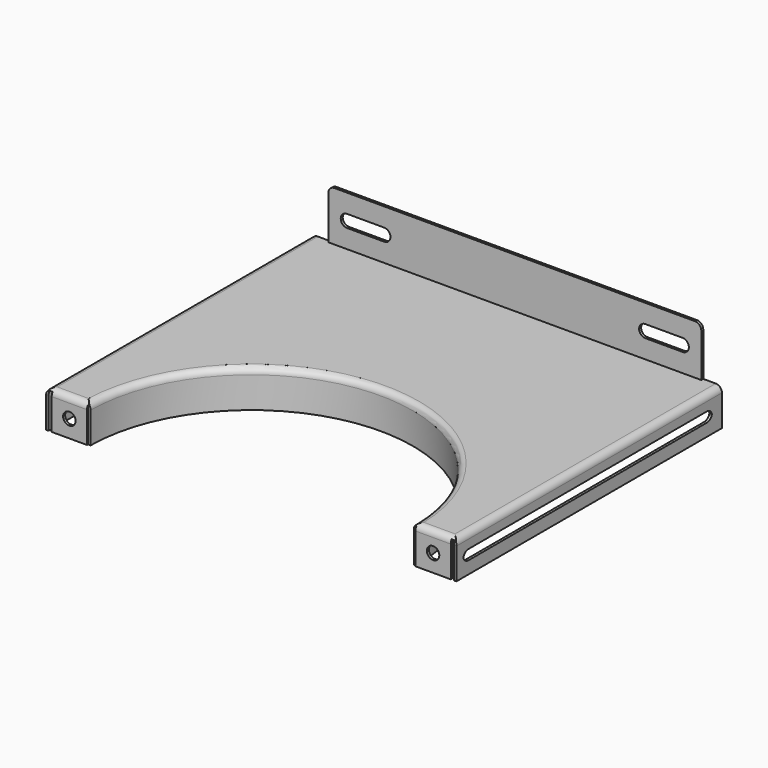
from build123d import *

# Parameters (mm, degrees)
F1_DEPTH       = 267
F2_W           = 250
F2_H           = 8
F3_DEPTH       = 5
F4_R           = 130
F5_DEPTH       = 12.5
F6_W           = 150
F6_H           = 40
F7_DEPTH       = 2
F8_W           = 40
F8_H           = 10
F9_DEPTH       = 12.5
F10_F1_R       = 5
F10_F2_R       = 5
F10_F3_R       = 4.9999
F10_F4_R       = 4.9999
F10_2_T1_DEPTH = 35
F11_W          = 28.4319519997
F11_H          = 28
F12_DEPTH      = 2
F13_R          = 5
F14_DEPTH      = 5
F17_T1_DEPTH   = 27
F17_T3_DEPTH   = 292
F17_T5_DEPTH   = 60
F20_DEPTH      = 28
F21_T2_ANGLE   = 186.62682558


# Not quite as in the source:
# - a fillet or chamfer that OpenCascade refuses, or shapes differently, is made with other operations: its cross-section is extruded or revolved along the edge and cut away or added
# - a fillet or chamfer is up to 0.001 mm smaller than in the source, because OpenCascade refuses the exact size


with BuildPart() as f1:
    # F0 (on Front) → F1 (new body)
    with BuildSketch(Plane.XZ):
        Polygon((-165, -30), (-163, -30), (-163, -2), (0, -2), (0, 0), (-165, 0), align=None)
    extrude(amount=F1_DEPTH)


with BuildPart() as f3:
    # F2 (on face) → F3 (new body, symmetric)
    with BuildSketch(Plane(origin=(-165, 0, 0), x_dir=(0, -1, 0), z_dir=(-1, 0, 0))):
        with Locations((135, -16)):
            Rectangle(F2_W, F2_H)
    extrude(amount=F3_DEPTH, both=True)

    # F10#2: fillet of radius 5 on 4 edges, made by hand

    # F10_2_s2 → F10_2_t1 (cut)
    with BuildSketch(Plane.YZ.offset(-182.5)):
        with BuildLine():
            ThreePointArc((-15, -12), (-11.4644660941, -13.4644660941), (-10, -17))
            Line((-10, -17), (-10, -12))
            Line((-10, -12), (-15, -12))
        make_face()
        with BuildLine():
            ThreePointArc((-15, -20), (-11.4644660941, -18.5355339059), (-10, -15))
            Line((-10, -15), (-10, -20))
            Line((-10, -20), (-15, -20))
        make_face()
        with BuildLine():
            ThreePointArc((-260, -15), (-258.5355339059, -18.5355339059), (-255, -20))
            Line((-255, -20), (-260, -20))
            Line((-260, -20), (-260, -15))
        make_face()
        with BuildLine():
            ThreePointArc((-255, -12), (-258.5355339059, -13.4644660941), (-260, -17))
            Line((-260, -17), (-260, -12))
            Line((-260, -12), (-255, -12))
        make_face()
    extrude(amount=F10_2_T1_DEPTH, mode=Mode.SUBTRACT)


with BuildPart() as f5:
    # F4 (on face) → F5 (new body, symmetric)
    with BuildSketch(Plane.XY):
        with Locations((0, -267)):
            Circle(F4_R)
    extrude(amount=F5_DEPTH, both=True)


with BuildPart() as f7:
    # F6 (on face) → F7 (new body)
    with BuildSketch(Plane(origin=(0, 0, 0), x_dir=(-1, 0, 0), z_dir=(0, 1, 0))):
        with Locations((75, 20)):
            Rectangle(F6_W, F6_H)
    extrude(amount=-F7_DEPTH)


with BuildPart() as f9:
    # F8 (on face) → F9 (new body, symmetric)
    with BuildSketch(Plane.XZ.offset(2)):
        with Locations((-120, 20)):
            Rectangle(F8_W, F8_H)
    extrude(amount=F9_DEPTH, both=True)

    # F10: fillet of radius 5 on 4 edges, made by hand

    # F10_f1
    f10_f1_edges = [f9.edges().sort_by_distance(p)[0] for p in [
        (-140, -2, 25),
    ]]
    fillet(f10_f1_edges, radius=F10_F1_R)

    # F10_f2
    f10_f2_edges = [f9.edges().sort_by_distance(p)[0] for p in [
        (-100, -2, 25),
    ]]
    fillet(f10_f2_edges, radius=F10_F2_R)

    # F10_f3 (radius 5 in the source; OpenCascade refuses exactly that, so slightly less here)
    f10_f3_edges = [f9.edges().sort_by_distance(p)[0] for p in [
        (-100, -2, 15),
    ]]
    fillet(f10_f3_edges, radius=F10_F3_R)

    # F10_f4 (radius 5 in the source; OpenCascade refuses exactly that, so slightly less here)
    f10_f4_edges = [f9.edges().sort_by_distance(p)[0] for p in [
        (-140, -2, 15),
    ]]
    fillet(f10_f4_edges, radius=F10_F4_R)


with BuildPart() as f12:
    # F11 (on face) → F12 (new body)
    with BuildSketch(Plane.XZ.offset(267)):
        with Locations((-146.2773531675, -16)):
            Rectangle(F11_W, F11_H)
    extrude(amount=-F12_DEPTH)


with BuildPart() as f14:
    # F13 (on face) → F14 (new body, symmetric)
    with BuildSketch(Plane.XZ.offset(267)):
        with Locations((-146.2773531675, -16)):
            Circle(F13_R)
    extrude(amount=F14_DEPTH, both=True)


with BuildPart() as f1_1:
    add(f1.part)

    # F15: union F7, F12
    add(f7.part)
    add(f12.part)

    # F16: cut F9, F3, F5, F14
    add(f9.part, mode=Mode.SUBTRACT)
    add(f3.part, mode=Mode.SUBTRACT)
    add(f5.part, mode=Mode.SUBTRACT)
    add(f14.part, mode=Mode.SUBTRACT)

    # F17: fillet of radius 5 on 3 edges, made by hand

    # F17_s2 → F17_t1 (cut)
    with BuildSketch(Plane.XZ.offset(-12.5)):
        with BuildLine():
            ThreePointArc((-150, 35), (-148.5355339059, 38.5355339059), (-145, 40))
            Line((-145, 40), (-150, 40))
            Line((-150, 40), (-150, 35))
        make_face()
    extrude(amount=F17_T1_DEPTH, mode=Mode.SUBTRACT)

    # F17_s4 → F17_t3 (cut)
    with BuildSketch(Plane.XZ.offset(-12.5)):
        with BuildLine():
            ThreePointArc((-165, -5), (-163.5355339059, -1.4644660941), (-160, 0))
            Line((-160, 0), (-165, 0))
            Line((-165, 0), (-165, -5))
        make_face()
    extrude(amount=F17_T3_DEPTH, mode=Mode.SUBTRACT)

    # F17_s6 → F17_t5 (cut)
    with BuildSketch(Plane.YZ.offset(-177.5)):
        with BuildLine():
            ThreePointArc((-267, -5), (-265.5355339059, -1.4644660941), (-262, 0))
            Line((-262, 0), (-267, 0))
            Line((-267, 0), (-267, -5))
        make_face()
    extrude(amount=F17_T5_DEPTH, mode=Mode.SUBTRACT)

    # F18: F1 across plane


with BuildPart() as f1_2:
    add(f1_1.part)
    add(f1_1.part.mirror(Plane.YZ))

    # F19 (on face) → F20 (join)
    with BuildSketch(Plane(origin=(0, 0, -2), x_dir=(1, 0, 0), z_dir=(0, 0, -1))):
        with BuildLine():
            ThreePointArc((129.9961537893, 266), (0, 137), (-129.9961537893, 266))
            Line((-129.9961537893, 266), (-131.9962120669, 266))
            ThreePointArc((-131.9962120669, 266), (0, 135), (131.9962120669, 266))
            Line((131.9962120669, 266), (129.9961537893, 266))
        make_face()
    extrude(amount=F20_DEPTH)

    # F21: fillet of radius 5 on 1 edges, made by hand

    # F21_s1 → F21_t2 (revolve, cut)
    with BuildSketch(Plane(origin=(15.4061976699, -266.1080656422, 0), x_dir=(0, 0, 1), z_dir=(0.0577977346, -0.9983283137, 0))):
        with BuildLine():
            ThreePointArc((0, 150.4319951252), (-1.4644660941, 146.8964612192), (-5, 145.4319951252))
            Line((-5, 145.4319951252), (0, 145.4319951252))
            Line((0, 145.4319951252), (0, 150.4319951252))
        make_face()
    revolve(axis=Axis((0, -267, 0), (0, 0, -1)), revolution_arc=F21_T2_ANGLE, mode=Mode.SUBTRACT)


solid = f1_2.part
